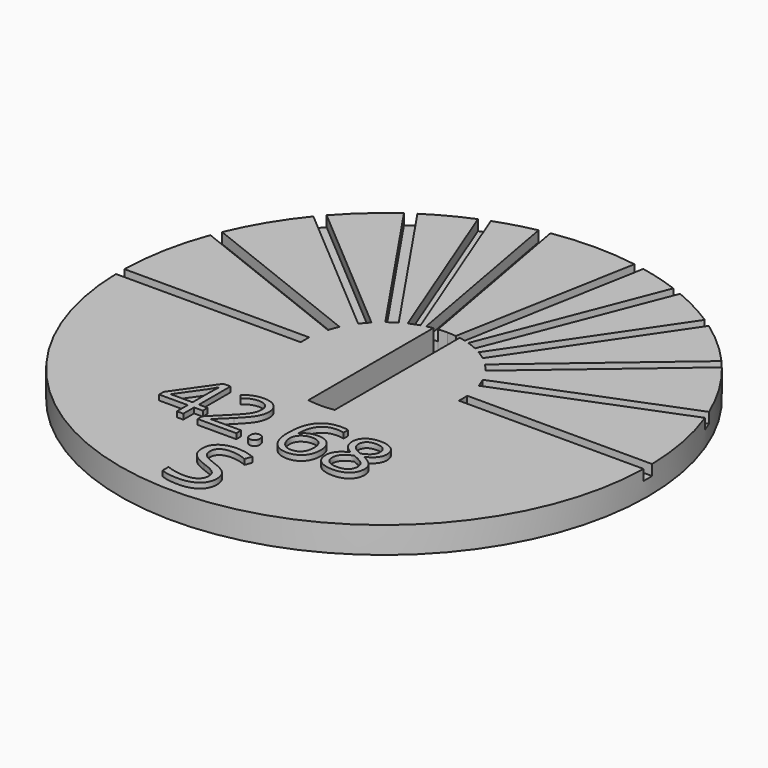
from build123d import *

# Parameters (mm, degrees)
F0_R         = 50
F1_DEPTH     = 5
F3_DEPTH     = 2
F5_TEXT_SIZE = 17.674675504
F6_DEPTH     = 1
F7_TEXT_SIZE = 15.5878950253
F8_DEPTH     = 1
F10_DEPTH    = 5.001


# Not quite as in the source:
# - a feature names something its author has since deleted; it is built from what else it names
# - Text() gives the source's letters only with a copy of the font that has no kerning and outlines rounded to 1/6400 em; it was checked with that copy


with BuildPart() as f1:
    # F0 (on Top) → F1 (new body)
    with BuildSketch(Plane.XY):
        Circle(F0_R)
    extrude(amount=F1_DEPTH)

    # F2 (on face) → F3 (cut)
    with BuildSketch(Plane.XY.offset(5)):
        with BuildLine():
            Line((-49.9899989998, -1), (-14.9666295471, -1))
            ThreePointArc((-14.9666295471, -1), (-15, 0), (-14.9666295471, 1))
            Line((-14.9666295471, 1), (-49.9899989998, 1))
            ThreePointArc((-49.9899989998, 1), (-50, 0), (-49.9899989998, -1))
        make_face()
        with BuildLine():
            Line((-46.8567924508, 17.4482377684), (-14.286140802, 4.5723277426))
            ThreePointArc((-14.286140802, 4.5723277426), (-13.9495366199, 5.5145650862), (-13.5508654572, 6.4322659586))
            Line((-13.5508654572, 6.4322659586), (-46.121517106, 19.3081759843))
            ThreePointArc((-46.121517106, 19.3081759843), (-46.4984553996, 18.3818836208), (-46.8567924508, 17.4482377684))
        make_face()
        with BuildLine():
            Line((-38.7063730379, 31.6514878994), (-12.0426607308, 8.9428363801))
            ThreePointArc((-12.0426607308, 8.9428363801), (-11.4196803693, 9.7257853288), (-10.7458893537, 10.4654604294))
            Line((-10.7458893537, 10.4654604294), (-37.4096016608, 33.1741119487))
            ThreePointArc((-37.4096016608, 33.1741119487), (-38.0656012311, 32.4192844294), (-38.7063730379, 31.6514878994))
        make_face()
        with BuildLine():
            Line((-28.8757798386, 40.8189825781), (-9.2251307642, 11.8278046308))
            ThreePointArc((-9.2251307642, 11.8278046308), (-8.416087336, 12.4165000685), (-7.5695974217, 12.9499496089))
            Line((-7.5695974217, 12.9499496089), (-27.2202464962, 41.9411275562))
            ThreePointArc((-27.2202464962, 41.9411275562), (-28.0536244535, 41.3883335618), (-28.8757798386, 40.8189825781))
        make_face()
        with BuildLine():
            Line((-19.1470642134, 46.1886342297), (-6.3849254233, 13.5732356989))
            ThreePointArc((-6.3849254233, 13.5732356989), (-5.4658385199, 13.968701059), (-4.5224319488, 14.3020141682))
            Line((-4.5224319488, 14.3020141682), (-17.2845707388, 46.9174126991))
            ThreePointArc((-17.2845707388, 46.9174126991), (-18.2194617329, 46.5623368632), (-19.1470642134, 46.1886342297))
        make_face()
        with BuildLine():
            ThreePointArc((-3.6599515538, 14.5466406646), (-2.6820332267, 14.758275569), (-1.6921814779, 14.9042450948))
            Line((-1.6921814779, 14.9042450948), (-7.9544375169, 49.3632142773))
            ThreePointArc((-7.9544375169, 49.3632142773), (-8.9401107558, 49.1942518967), (-9.9222075928, 49.0056098471))
            Line((-9.9222075928, 49.0056098471), (-3.6599515538, 14.5466406646))
        make_face()
        with BuildLine():
            ThreePointArc((1.6921814779, 14.9042450948), (2.6820332267, 14.758275569), (3.6599515538, 14.5466406646))
            Line((3.6599515538, 14.5466406646), (9.9222075928, 49.0056098471))
            ThreePointArc((9.9222075928, 49.0056098471), (8.9401107558, 49.1942518967), (7.9544375169, 49.3632142773))
            Line((7.9544375169, 49.3632142773), (1.6921814779, 14.9042450948))
        make_face()
        with BuildLine():
            ThreePointArc((4.5224319488, 14.3020141682), (5.4658385199, 13.968701059), (6.3849254233, 13.5732356989))
            Line((6.3849254233, 13.5732356989), (19.1470642134, 46.1886342297))
            ThreePointArc((19.1470642134, 46.1886342297), (18.2194617329, 46.5623368632), (17.2845707388, 46.9174126991))
            Line((17.2845707388, 46.9174126991), (4.5224319488, 14.3020141682))
        make_face()
        with BuildLine():
            ThreePointArc((7.5695974217, 12.9499496089), (8.416087336, 12.4165000685), (9.2251307642, 11.8278046308))
            Line((9.2251307642, 11.8278046308), (28.8757798386, 40.8189825781))
            ThreePointArc((28.8757798386, 40.8189825781), (28.0536244535, 41.3883335618), (27.2202464962, 41.9411275562))
            Line((27.2202464962, 41.9411275562), (7.5695974217, 12.9499496089))
        make_face()
        with BuildLine():
            ThreePointArc((10.7458893537, 10.4654604294), (11.4196803693, 9.7257853288), (12.0426607308, 8.9428363801))
            Line((12.0426607308, 8.9428363801), (38.7063730379, 31.6514878994))
            ThreePointArc((38.7063730379, 31.6514878994), (38.0656012311, 32.4192844294), (37.4096016608, 33.1741119487))
            Line((37.4096016608, 33.1741119487), (10.7458893537, 10.4654604294))
        make_face()
        with BuildLine():
            ThreePointArc((13.5508654572, 6.4322659586), (13.9495366199, 5.5145650862), (14.286140802, 4.5723277426))
            Line((14.286140802, 4.5723277426), (46.8567924508, 17.4482377684))
            ThreePointArc((46.8567924508, 17.4482377684), (46.4984553996, 18.3818836208), (46.121517106, 19.3081759843))
            Line((46.121517106, 19.3081759843), (13.5508654572, 6.4322659586))
        make_face()
        with BuildLine():
            ThreePointArc((14.9666295471, 1), (14.9916550655, 0.5002783193), (15, 0))
            ThreePointArc((15, 0), (14.9916550655, -0.5002783193), (14.9666295471, -1))
            Line((14.9666295471, -1), (49.9899989998, -1))
            ThreePointArc((49.9899989998, -1), (49.9974996874, -0.5000250044), (50, 0))
            ThreePointArc((50, 0), (49.9974996874, 0.5000250044), (49.9899989998, 1))
            Line((49.9899989998, 1), (14.9666295471, 1))
        make_face()
    extrude(amount=-F3_DEPTH, mode=Mode.SUBTRACT)

    # F5 (on face) → F6 (join)
    with BuildSketch(Plane.XY.offset(5)):
        with Locations((-5, -47.7257663629)):
            Text('S', F5_TEXT_SIZE, font='Open Sans', text_align=(TextAlign.LEFT, TextAlign.BOTTOM))
    extrude(amount=F6_DEPTH)

    # F7 (on face) → F8 (join)
    with BuildSketch(Plane.XY.offset(5)):
        with Locations((-20, -31.2232844182)):
            Text('42.68', F7_TEXT_SIZE, font='Open Sans', text_align=(TextAlign.LEFT, TextAlign.BOTTOM))
    extrude(amount=F8_DEPTH)

    # F9 (on face) → F10 (cut, through all)
    with BuildSketch(Plane.XY.offset(5)):
        with BuildLine():
            ThreePointArc((-2.5, -14.7901994577), (-1.2543939042, -14.9474578418), (0, -15))
            ThreePointArc((0, -15), (1.2543939042, -14.9474578418), (2.5, -14.7901994577))
            Line((2.5, -14.7901994577), (2.5, 14.7901994577))
            ThreePointArc((2.5, 14.7901994577), (2.0968662303, 14.8527153077), (1.6921814779, 14.9042450948))
            ThreePointArc((1.6921814779, 14.9042450948), (0.847444269, 14.9760421411), (0, 15))
            ThreePointArc((0, 15), (-0.847444269, 14.9760421411), (-1.6921814779, 14.9042450948))
            ThreePointArc((-1.6921814779, 14.9042450948), (-2.0968662303, 14.8527153077), (-2.5, 14.7901994577))
            Line((-2.5, 14.7901994577), (-2.5, -14.7901994577))
        make_face()
    extrude(amount=-F10_DEPTH, mode=Mode.SUBTRACT)


solid = f1.part
